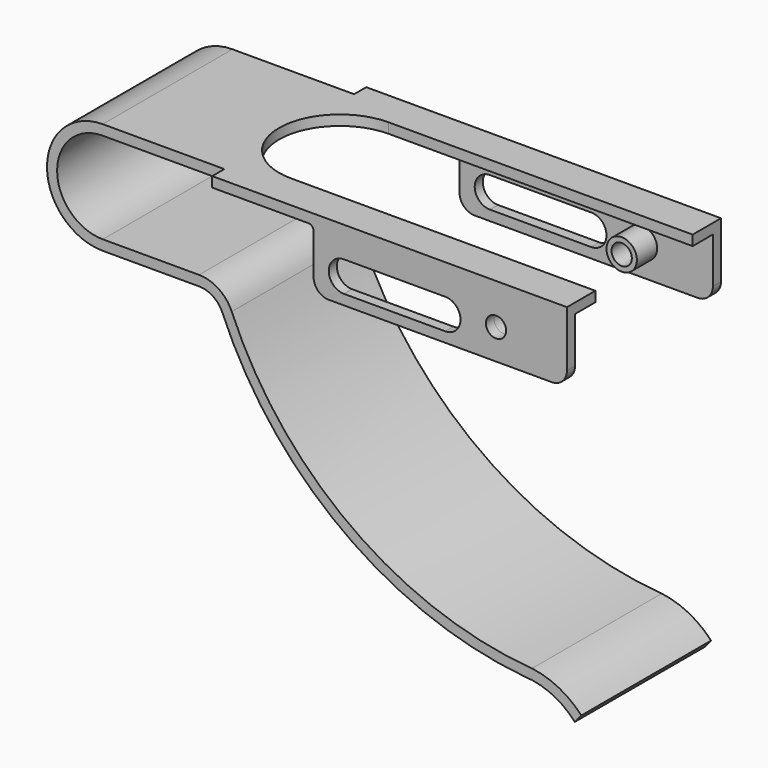
from build123d import *

# Parameters (mm, degrees)
F1_DEPTH  = 16
F2_W      = 70
F2_H      = 3
F3_DEPTH  = 2
F4_W      = 50
F4_H      = 14
F5_DEPTH  = 2
F6_R      = 1
F9_DEPTH  = 2
F11_DEPTH = 38.001
F13_D     = 4
F14_R     = 3
F14_R_2   = 2
F15_DEPTH = 5
F16_R     = 3


# Not quite as in the source:
# - a pattern or mirror of a feature is missing from the dataset's text; its kind, count and spacing are read off the source's solid


with BuildPart() as f1:
    # F0 (on Front) → F1 (new body)
    with BuildSketch(Plane.XZ):
        with BuildLine():
            Line((94, 11), (0, 11))
            ThreePointArc((0, 11), (-11, 0), (0, -11))
            Line((0, -11), (19, -11))
            ThreePointArc((19, -11), (21.7681124643, -11.8361612201), (23.6103896104, -14.064978646))
            ThreePointArc((23.6103896104, -14.064978646), (47.381548553, -44.2322797447), (83.2800086179, -57.8863860143))
            ThreePointArc((83.2800086179, -57.8863860143), (88.6838234672, -59.2161173312), (93.142692854, -62.5459647892))
            Line((93.142692854, -62.5459647892), (94.4399113384, -61))
            ThreePointArc((94.4399113384, -61), (90.012513527, -57.6415445278), (84.7034264019, -56))
            ThreePointArc((84.7034264019, -56), (49.0672193413, -42.9854179344), (25.4545454545, -13.2909701044))
            ThreePointArc((25.4545454545, -13.2909701044), (22.87535745, -10.1706257081), (19, -9))
            Line((19, -9), (0, -9))
            ThreePointArc((0, -9), (-9, 0), (0, 9))
            Line((0, 9), (94, 9))
            Line((94, 9), (94, 11))
        make_face()
    extrude(amount=F1_DEPTH)

    # F2 (on face) → F3 (join)
    with BuildSketch(Plane.XY.offset(11)):
        with Locations((59, -17.5)):
            Rectangle(F2_W, F2_H)
    extrude(amount=-F3_DEPTH)

    # F4 (on face) → F5 (join)
    with BuildSketch(Plane.XZ.offset(19)):
        with Locations((69, 4)):
            Rectangle(F4_W, F4_H)
    extrude(amount=-F5_DEPTH)

    # F6
    f6_edges = [f1.edges().sort_by_distance(p)[0] for p in [
        (44, -18, 9),
    ]]
    fillet(f6_edges, radius=F6_R)

    # F7: F1 across plane


with BuildPart() as f1_1:
    add(f1.part)
    add(f1.part.mirror(Plane.XZ))

    # F8 (on face) → F9 (cut)
    with BuildSketch(Plane.XY.offset(11)):
        with BuildLine():
            Line((94, 12), (34, 12))
            ThreePointArc((34, 12), (22, 0), (34, -12))
            Line((34, -12), (94, -12))
            Line((94, -12), (94, 12))
        make_face()
    extrude(amount=-F9_DEPTH, mode=Mode.SUBTRACT)

    # F10 (on face) → F11 (cut, through all)
    with BuildSketch(Plane.XZ.offset(19)):
        with BuildLine():
            ThreePointArc((50, 5), (47, 2), (50, -1))
            Line((50, -1), (70, -1))
            ThreePointArc((70, -1), (73, 2), (70, 5))
            Line((70, 5), (50, 5))
        make_face()
    extrude(amount=-F11_DEPTH, mode=Mode.SUBTRACT)

    # F13 (through all)
    with Locations(Plane.XZ.offset(19)):
        with Locations((80, 3)):
            Hole(F13_D / 2)

    # F14 (on face) → F15 (join)
    with BuildSketch(Plane(origin=(0, -17, 0), x_dir=(-1, 0, 0), z_dir=(0, 1, 0))):
        with Locations((-80, 3)):
            Circle(F14_R)
        with Locations((-80, 3)):
            Circle(F14_R_2, mode=Mode.SUBTRACT)
    f15 = extrude(amount=F15_DEPTH)

    # F15_copies: F15 across plane
    add(f15.mirror(Plane.ZX))

    # F16
    f16_edges = [f1_1.edges().sort_by_distance(p)[0] for p in [
        (94, -18, -3),
        (44, -18, -3),
        (94, 18, -3),
        (44, 18, -3),
    ]]
    fillet(f16_edges, radius=F16_R)


solid = f1_1.part
